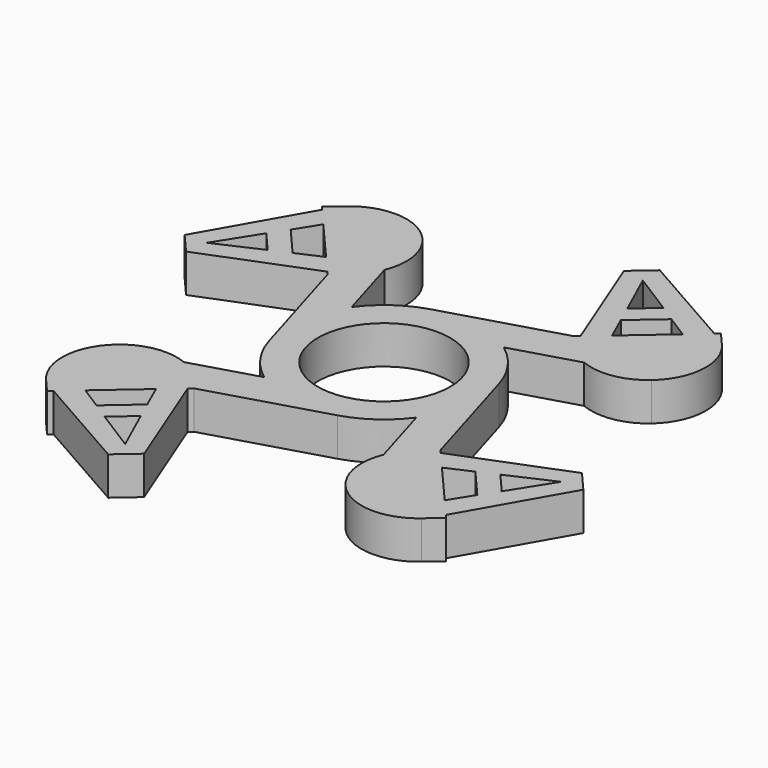
from build123d import *

# Parameters (mm, degrees)
F0_TEXT_SIZE = 25.2370109708
F0_R         = 11
F1_DEPTH     = 6.35


# Not quite as in the source:
# - Text() gives the source's letters only with a copy of the font that has no kerning and outlines rounded to 1/6400 em; it was checked with that copy


with BuildPart() as f1:
    # F0 (on Top) → F1 (new body)
    with BuildSketch(Plane.XY):
        with BuildLine():
            Line((31.172129121, 31.206713878), (29.0931613351, 33.6064050968))
            Line((29.0931613351, 33.6064050968), (28.4562323214, 33.0546028936))
            Line((28.4562323214, 33.0546028936), (25.3447303976, 30.3589592979))
            Line((25.3447303976, 30.3589592979), (18.4064387512, 24.3479839237))
            Line((18.4064387512, 24.3479839237), (15.2949368273, 21.6523403281))
            Line((15.2949368273, 21.6523403281), (14.6950140226, 21.1325983816))
            Line((14.6950140226, 21.1325983816), (16.7739818085, 18.7329071628))
            ThreePointArc((16.7739818085, 18.7329071628), (18.3951921729, 17.2488607021), (20.3133977767, 16.175918856))
            ThreePointArc((20.3133977767, 16.175918856), (25.4884464803, 15.5661295885), (30.2099588223, 17.7707368642))
            ThreePointArc((30.2099588223, 17.7707368642), (33.4737259231, 24.2894533776), (31.172129121, 31.206713878))
        make_face()
        with Locations(Location((15.2949368273, 21.6523403281), (0, 0, 40.9039562418))):
            Text('A', F0_TEXT_SIZE, font='Open Sans', font_style=FontStyle.BOLD, text_align=(TextAlign.LEFT, TextAlign.BOTTOM))
        with BuildLine():
            Line((9.5057851937, 12.9694428505), (20.3133977767, 16.175918856))
            ThreePointArc((20.3133977767, 16.175918856), (18.3951921729, 17.2488607021), (16.7739818085, 18.7329071628))
            Line((16.7739818085, 18.7329071628), (14.6950140226, 21.1325983816))
            Line((14.6950140226, 21.1325983816), (-4.5736741572, 15.4158329228))
            ThreePointArc((-4.5736741572, 15.4158329228), (2.752750609, 15.8426249114), (9.5057851937, 12.9694428505))
        make_face()
        with BuildLine():
            ThreePointArc((15.4158329228, 4.5736741572), (13.1489161292, 9.2559388841), (9.5057851937, 12.9694428505))
            ThreePointArc((9.5057851937, 12.9694428505), (2.752750609, 15.8426249114), (-4.5736741572, 15.4158329228))
            ThreePointArc((-4.5736741572, 15.4158329228), (-9.2559388841, 13.1489161292), (-12.9694428505, 9.5057851937))
            ThreePointArc((-12.9694428505, 9.5057851937), (-15.8426249114, 2.752750609), (-15.4158329228, -4.5736741572))
            ThreePointArc((-15.4158329228, -4.5736741572), (-13.1489161292, -9.2559388841), (-9.5057851937, -12.9694428505))
            ThreePointArc((-9.5057851937, -12.9694428505), (-2.752750609, -15.8426249114), (4.5736741572, -15.4158329228))
            ThreePointArc((4.5736741572, -15.4158329228), (9.2559388841, -13.1489161292), (12.9694428505, -9.5057851937))
            ThreePointArc((12.9694428505, -9.5057851937), (15.2825888029, -5.0008878694), (16.08, 0))
            ThreePointArc((16.08, 0), (15.9130919905, 2.3108230786), (15.4158329228, 4.5736741572))
        make_face()
        Circle(F0_R, mode=Mode.SUBTRACT)
        with BuildLine():
            Line((21.1325983816, -14.6950140226), (15.4158329228, 4.5736741572))
            ThreePointArc((15.4158329228, 4.5736741572), (15.9130919905, 2.3108230786), (16.08, 0))
            ThreePointArc((16.08, 0), (15.2825888029, -5.0008878694), (12.9694428505, -9.5057851937))
            Line((12.9694428505, -9.5057851937), (16.175918856, -20.3133977767))
            ThreePointArc((16.175918856, -20.3133977767), (17.2488607021, -18.3951921729), (18.7329071628, -16.7739818085))
            Line((18.7329071628, -16.7739818085), (21.1325983816, -14.6950140226))
        make_face()
        with BuildLine():
            Line((21.6523403281, -15.2949368273), (21.1325983816, -14.6950140226))
            Line((21.1325983816, -14.6950140226), (18.7329071628, -16.7739818085))
            ThreePointArc((18.7329071628, -16.7739818085), (17.2488607021, -18.3951921729), (16.175918856, -20.3133977767))
            ThreePointArc((16.175918856, -20.3133977767), (15.5661295885, -25.4884464803), (17.7707368642, -30.2099588223))
            ThreePointArc((17.7707368642, -30.2099588223), (24.2894533776, -33.4737259231), (31.206713878, -31.172129121))
            Line((31.206713878, -31.172129121), (33.6064050968, -29.0931613351))
            Line((33.6064050968, -29.0931613351), (33.0546028936, -28.4562323214))
            Line((33.0546028936, -28.4562323214), (30.3589592979, -25.3447303976))
            Line((30.3589592979, -25.3447303976), (24.3479839237, -18.4064387512))
            Line((24.3479839237, -18.4064387512), (21.6523403281, -15.2949368273))
        make_face()
        with BuildLine():
            ThreePointArc((-15.4158329228, -4.5736741572), (-15.8426249114, 2.752750609), (-12.9694428505, 9.5057851937))
            Line((-12.9694428505, 9.5057851937), (-16.175918856, 20.3133977767))
            ThreePointArc((-16.175918856, 20.3133977767), (-17.2488607021, 18.3951921729), (-18.7329071628, 16.7739818085))
            Line((-18.7329071628, 16.7739818085), (-21.1325983816, 14.6950140226))
            Line((-21.1325983816, 14.6950140226), (-15.4158329228, -4.5736741572))
        make_face()
        with Locations(Location((21.6523403281, -15.2949368273), (0, 0, -49.0960437582))):
            Text('A', F0_TEXT_SIZE, font='Open Sans', font_style=FontStyle.BOLD, text_align=(TextAlign.LEFT, TextAlign.BOTTOM))
        with BuildLine():
            ThreePointArc((-18.7329071628, 16.7739818085), (-17.2488607021, 18.3951921729), (-16.175918856, 20.3133977767))
            ThreePointArc((-16.175918856, 20.3133977767), (-15.5661295885, 25.4884464803), (-17.7707368642, 30.2099588223))
            ThreePointArc((-17.7707368642, 30.2099588223), (-24.2894533776, 33.4737259231), (-31.206713878, 31.172129121))
            Line((-31.206713878, 31.172129121), (-33.6064050968, 29.0931613351))
            Line((-33.6064050968, 29.0931613351), (-33.0546028936, 28.4562323214))
            Line((-33.0546028936, 28.4562323214), (-30.3589592979, 25.3447303976))
            Line((-30.3589592979, 25.3447303976), (-24.3479839237, 18.4064387512))
            Line((-24.3479839237, 18.4064387512), (-21.6523403281, 15.2949368273))
            Line((-21.6523403281, 15.2949368273), (-21.1325983816, 14.6950140226))
            Line((-21.1325983816, 14.6950140226), (-18.7329071628, 16.7739818085))
        make_face()
        with BuildLine():
            Line((-14.6950140226, -21.1325983816), (4.5736741572, -15.4158329228))
            ThreePointArc((4.5736741572, -15.4158329228), (-2.752750609, -15.8426249114), (-9.5057851937, -12.9694428505))
            Line((-9.5057851937, -12.9694428505), (-20.3133977767, -16.175918856))
            ThreePointArc((-20.3133977767, -16.175918856), (-18.3951921729, -17.2488607021), (-16.7739818085, -18.7329071628))
            Line((-16.7739818085, -18.7329071628), (-14.6950140226, -21.1325983816))
        make_face()
        with BuildLine():
            Line((-15.2949368273, -21.6523403281), (-14.6950140226, -21.1325983816))
            Line((-14.6950140226, -21.1325983816), (-16.7739818085, -18.7329071628))
            ThreePointArc((-16.7739818085, -18.7329071628), (-18.3951921729, -17.2488607021), (-20.3133977767, -16.175918856))
            ThreePointArc((-20.3133977767, -16.175918856), (-25.4884464803, -15.5661295885), (-30.2099588223, -17.7707368642))
            ThreePointArc((-30.2099588223, -17.7707368642), (-33.4737259231, -24.2894533776), (-31.172129121, -31.206713878))
            Line((-31.172129121, -31.206713878), (-29.0931613351, -33.6064050968))
            Line((-29.0931613351, -33.6064050968), (-28.4562323214, -33.0546028936))
            Line((-28.4562323214, -33.0546028936), (-25.3447303976, -30.3589592979))
            Line((-25.3447303976, -30.3589592979), (-18.4064387512, -24.3479839237))
            Line((-18.4064387512, -24.3479839237), (-15.2949368273, -21.6523403281))
        make_face()
        with Locations(Location((-21.6523403281, 15.2949368273), (0, 0, 130.9039562418))):
            Text('A', F0_TEXT_SIZE, font='Open Sans', font_style=FontStyle.BOLD, text_align=(TextAlign.LEFT, TextAlign.BOTTOM))
        with Locations(Location((-15.2949368273, -21.6523403281), (0, 0, -139.0960437582))):
            Text('A', F0_TEXT_SIZE, font='Open Sans', font_style=FontStyle.BOLD, text_align=(TextAlign.LEFT, TextAlign.BOTTOM))
    extrude(amount=F1_DEPTH)


solid = f1.part
